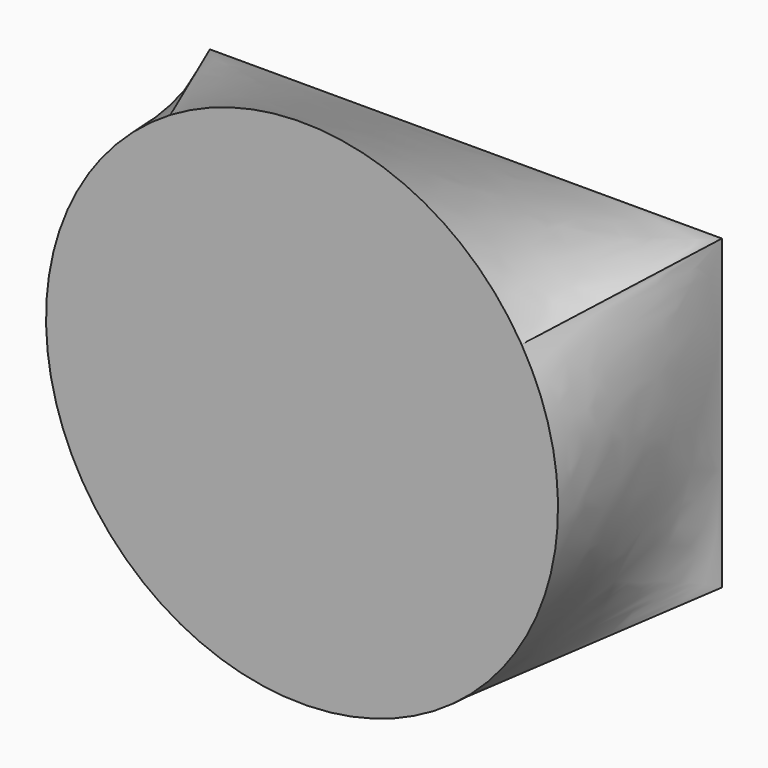
from build123d import *

# Parameters (mm, degrees)
F0_W = 127
F0_H = 76.2


# Not quite as in the source:
# - the arcs of a loft's sections are written as splines that run evenly, so that the points pair up as in the source's solid


with BuildPart() as f3:
    # F0 (on Front) → F3 section 0
    with BuildSketch(Plane.XZ):
        Rectangle(F0_W, F0_H)
    # F2 (on offset) → F3 section 1
    with BuildSketch(Plane.XZ.offset(50.8)):
        with BuildLine():
            add(Edge.make_bspline(
                [(54.4508007827, 32.6704804696), (52.3125228362, 36.2342770472), (49.8233031159, 39.5873887146), (44.2383956014, 45.7437124995), (41.142845905, 48.5467723897), (34.4642116327, 53.4952427339), (30.8812921992, 55.6405308272), (23.3655873388, 59.1909807904), (19.4329877526, 60.5960548685), (11.369036627, 62.6120426499), (7.2378844848, 63.222906504), (-1.0644197865, 63.6269588236), (-5.2353666247, 63.4201372982), (-13.4569711446, 62.1967266521), (-17.5074255309, 61.1801677826), (-25.3323786483, 58.3763091557), (-29.1066838921, 56.5890787293), (-32.6704804696, 54.4508007827)],
                knots=[0, 0, 0, 0, 0.125, 0.125, 0.25, 0.25, 0.375, 0.375, 0.5, 0.5, 0.625, 0.625, 0.75, 0.75, 0.875, 0.875, 1, 1, 1, 1], degree=3))
            add(Edge.make_bspline(
                [(-32.6704804696, 54.4508007827), (-36.2342770472, 52.3125228362), (-39.5873887146, 49.8233031159), (-45.7437124995, 44.2383956014), (-48.5467723897, 41.142845905), (-53.4952427339, 34.4642116327), (-55.6405308272, 30.8812921992), (-59.1909807904, 23.3655873388), (-60.5960548685, 19.4329877526), (-62.6120426499, 11.369036627), (-63.222906504, 7.2378844848), (-63.6269588236, -1.0644197865), (-63.4201372982, -5.2353666247), (-62.1967266521, -13.4569711446), (-61.1801677826, -17.5074255309), (-58.3763091557, -25.3323786483), (-56.5890787293, -29.1066838921), (-54.4508007827, -32.6704804696)],
                knots=[0, 0, 0, 0, 0.125, 0.125, 0.25, 0.25, 0.375, 0.375, 0.5, 0.5, 0.625, 0.625, 0.75, 0.75, 0.875, 0.875, 1, 1, 1, 1], degree=3))
            add(Edge.make_bspline(
                [(-54.4508007827, -32.6704804696), (-52.3125228362, -36.2342770472), (-49.8233031159, -39.5873887146), (-44.2383956014, -45.7437124995), (-41.142845905, -48.5467723897), (-34.4642116327, -53.4952427339), (-30.8812921992, -55.6405308272), (-23.3655873388, -59.1909807904), (-19.4329877526, -60.5960548685), (-11.369036627, -62.6120426499), (-7.2378844848, -63.222906504), (1.0644197865, -63.6269588236), (5.2353666247, -63.4201372982), (13.4569711446, -62.1967266521), (17.5074255309, -61.1801677826), (25.3323786483, -58.3763091557), (29.1066838921, -56.5890787293), (32.6704804696, -54.4508007827)],
                knots=[0, 0, 0, 0, 0.125, 0.125, 0.25, 0.25, 0.375, 0.375, 0.5, 0.5, 0.625, 0.625, 0.75, 0.75, 0.875, 0.875, 1, 1, 1, 1], degree=3))
            add(Edge.make_bspline(
                [(32.6704804696, -54.4508007827), (36.2342770472, -52.3125228362), (39.5873887146, -49.8233031159), (45.7437124995, -44.2383956014), (48.5467723897, -41.142845905), (53.4952427339, -34.4642116327), (55.6405308272, -30.8812921992), (59.1909807904, -23.3655873388), (60.5960548685, -19.4329877526), (62.6120426499, -11.369036627), (63.222906504, -7.2378844848), (63.6269588236, 1.0644197865), (63.4201372982, 5.2353666247), (62.1967266521, 13.4569711446), (61.1801677826, 17.5074255309), (58.3763091557, 25.3323786483), (56.5890787293, 29.1066838921), (54.4508007827, 32.6704804696)],
                knots=[0, 0, 0, 0, 0.125, 0.125, 0.25, 0.25, 0.375, 0.375, 0.5, 0.5, 0.625, 0.625, 0.75, 0.75, 0.875, 0.875, 1, 1, 1, 1], degree=3))
        make_face()
    loft(ruled=True)


solid = f3.part
